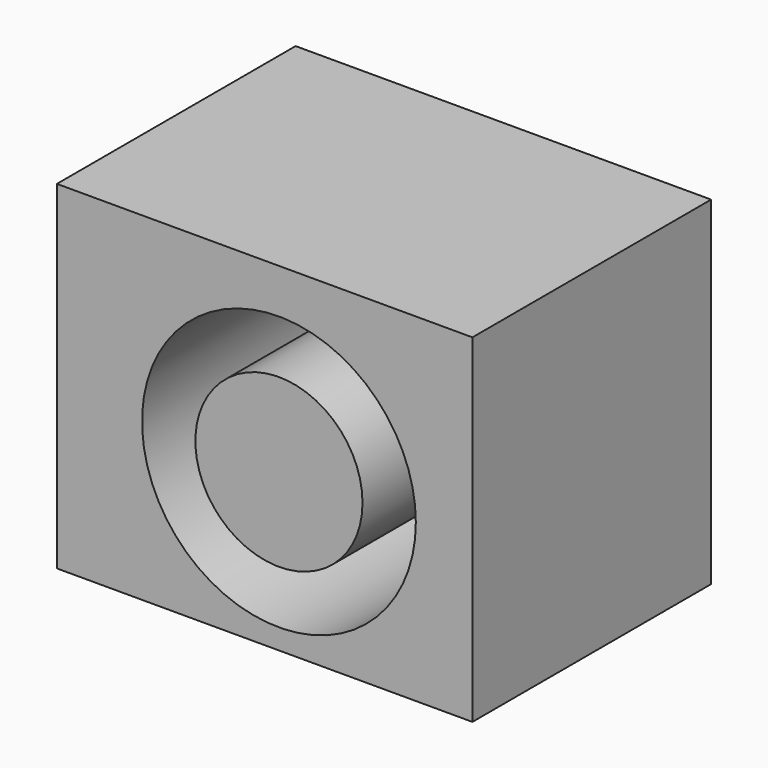
from build123d import *

# Parameters (mm, degrees)
F0_W     = 60.4875590652
F0_H     = 49.2861624807
F0_R     = 19.9281126129
F1_DEPTH = 43.434
F0_R_2   = 12.1657306008


# Not quite as in the source:
# - the program builds the solid bodies; features that only make, move or delete a surface that nothing else refers to are left out


with BuildPart() as f1:
    # F0 (on Front) → F1 (new body)
    with BuildSketch(Plane.XZ):
        with Locations((-2.0802589133, 1.7602192238)):
            Rectangle(F0_W, F0_H)
        Circle(F0_R, mode=Mode.SUBTRACT)
    extrude(amount=F1_DEPTH)


with BuildPart() as f1b:
    # F0 (on Front) → F1, piece 2 (new body)
    with BuildSketch(Plane.XZ):
        Circle(F0_R_2)
    extrude(amount=F1_DEPTH)


solid = Compound([f1.part, f1b.part])
